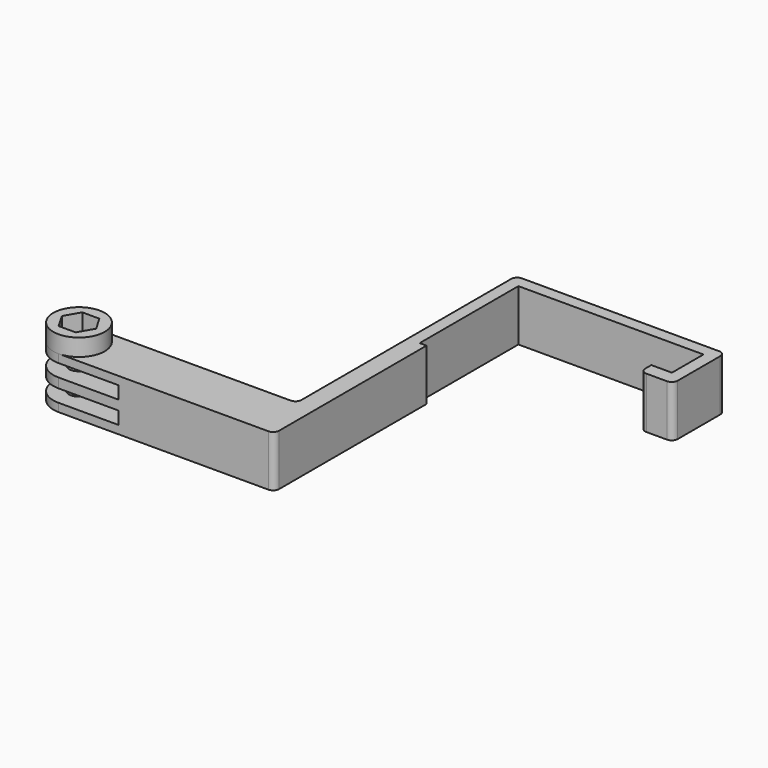
from build123d import *

# Parameters (mm, degrees)
F0_W      = 2
F0_H      = 10
F0_H_2    = 15
F1_DEPTH  = 15
F2_W      = 15
F2_H      = 15
F3_DEPTH  = 65
F5_DEPTH  = 25
F6_DEPTH  = 5
F7_R      = 2.875
F8_DEPTH  = 5
F9_DEPTH  = 25
F10_W     = 10
F10_H     = 3.7
F10_W_2   = 7.5
F11_DEPTH = 25
F12_W     = 30.5
F12_H     = 15
F13_DEPTH = 2
F14_R     = 1.75


with BuildPart() as f1:
    # F0 (on Top) → F1 (new body)
    with BuildSketch(Plane.XY):
        with Locations((-25.5, -71.0108693689)):
            Rectangle(F0_W, F0_H)
        Polygon((31, 3.9891306311), (-30, 3.9891306311), (-30, -91.0108693689), (-26.5, -91.0108693689), (-26.5, -76.0108693689), (-26.5, -66.0108693689), (-26.5, 0.4891306311), (27.5, 0.4891306311), (27.5, -11.0108693689), (21.5, -11.0108693689), (21.5, -15.0108693689), (31, -15.0108693689), align=None)
        with Locations((-25.5, -83.5108693689)):
            Rectangle(F0_W, F0_H_2)
    extrude(amount=F1_DEPTH)

    # F2 (on face) → F3 (join)
    with BuildSketch(Plane(origin=(-30, 0, 0), x_dir=(0, -1, 0), z_dir=(-1, 0, 0))):
        with Locations((83.5108693689, 7.5)):
            Rectangle(F2_W, F2_H)
    extrude(amount=F3_DEPTH)

    # F4 (on face) → F5 (cut)
    with BuildSketch(Plane.XY.offset(15)):
        with BuildLine():
            ThreePointArc((-95, -83.5108693689), (-92.8033008589, -78.20756851), (-87.5, -76.0108693689))
            Line((-87.5, -76.0108693689), (-95, -76.0108693689))
            Line((-95, -76.0108693689), (-95, -83.5108693689))
        make_face()
        with BuildLine():
            Line((-95, -91.0108693689), (-87.5, -91.0108693689))
            ThreePointArc((-87.5, -91.0108693689), (-92.8033008589, -88.8141702278), (-95, -83.5108693689))
            Line((-95, -83.5108693689), (-95, -91.0108693689))
        make_face()
    extrude(amount=-F5_DEPTH, mode=Mode.SUBTRACT)

    # F4 (on face) → F6 (join)
    with BuildSketch(Plane.XY.offset(15)):
        with BuildLine():
            ThreePointArc((-80, -83.5108693689), (-82.1966991411, -78.20756851), (-87.5, -76.0108693689))
            ThreePointArc((-87.5, -76.0108693689), (-92.8033008589, -78.20756851), (-95, -83.5108693689))
            ThreePointArc((-95, -83.5108693689), (-92.8033008589, -88.8141702278), (-87.5, -91.0108693689))
            ThreePointArc((-87.5, -91.0108693689), (-82.1966991411, -88.8141702278), (-80, -83.5108693689))
        make_face()
        with BuildLine():
            ThreePointArc((-84.625, -83.5108693689), (-87.5, -86.3858693689), (-90.375, -83.5108693689))
            ThreePointArc((-90.375, -83.5108693689), (-87.5, -80.6358693689), (-84.625, -83.5108693689))
        make_face(mode=Mode.SUBTRACT)
    extrude(amount=F6_DEPTH)

    # F7 (on face) → F8 (cut)
    with BuildSketch(Plane.XY.offset(20)):
        Polygon((-85, -79.18074235), (-90, -79.18074235), (-92.5, -83.5108693689), (-90, -87.8409963878), (-85, -87.8409963878), (-82.5, -83.5108693689), align=None)
        with Locations((-87.5, -83.5108693689)):
            Circle(F7_R, mode=Mode.SUBTRACT)
    extrude(amount=-F8_DEPTH, mode=Mode.SUBTRACT)

    # F4 (on face) → F9 (cut)
    with BuildSketch(Plane.XY.offset(15)):
        with BuildLine():
            ThreePointArc((-84.625, -83.5108693689), (-87.5, -80.6358693689), (-90.375, -83.5108693689))
            ThreePointArc((-90.375, -83.5108693689), (-87.5, -86.3858693689), (-84.625, -83.5108693689))
        make_face()
    extrude(amount=-F9_DEPTH, mode=Mode.SUBTRACT)

    # F10 (on face) → F11 (cut)
    with BuildSketch(Plane.XZ.offset(91.0108693689)):
        with Locations((-75, 10.75)):
            Rectangle(F10_W, F10_H)
        with Locations((-91.25, 10.75)):
            Rectangle(F10_W_2, F10_H)
        with Locations((-83.75, 10.75)):
            Rectangle(F10_W_2, F10_H)
        with Locations((-83.75, 4.25)):
            Rectangle(F10_W_2, F10_H)
        with Locations((-91.25, 4.25)):
            Rectangle(F10_W_2, F10_H)
        with Locations((-75, 4.25)):
            Rectangle(F10_W, F10_H)
    extrude(amount=-F11_DEPTH, mode=Mode.SUBTRACT)

    # F12 (on face) → F13 (join)
    with BuildSketch(Plane.YZ.offset(-26.5)):
        with Locations((-50.7608693689, 7.5)):
            Rectangle(F12_W, F12_H)
    extrude(amount=F13_DEPTH)

    # F14
    f14_edges = [f1.edges().sort_by_distance(p)[0] for p in [
        (-30, -76.010869, 7.5),
        (-30, 3.989131, 7.5),
        (31, 3.989131, 7.5),
        (31, -15.010869, 7.5),
        (21.5, -15.010869, 7.5),
        (-24.5, -91.010869, 7.5),
    ]]
    fillet(f14_edges, radius=F14_R)


solid = f1.part
